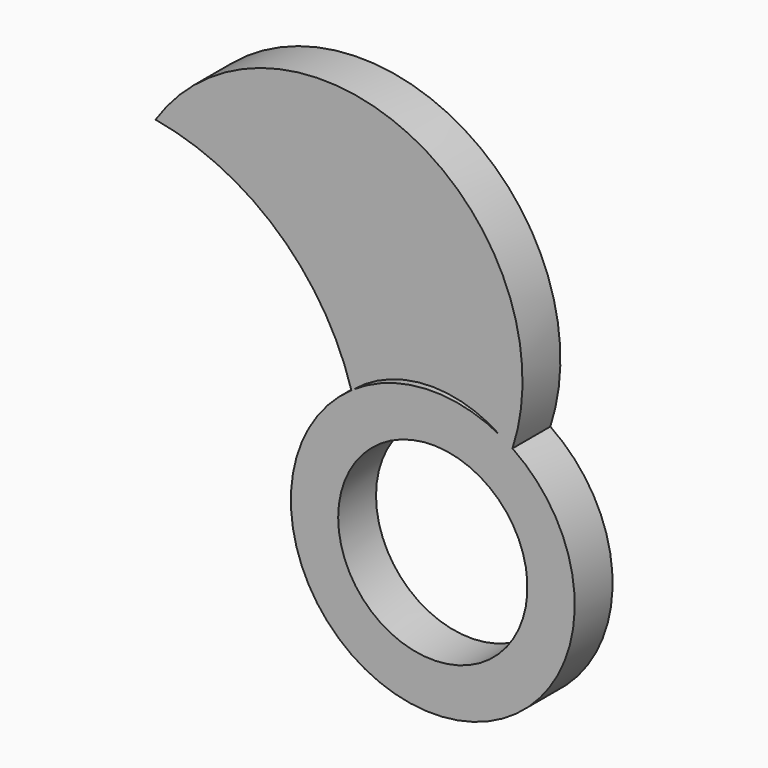
from build123d import *

# Parameters (mm, degrees)
F0_R     = 7.62
F1_DEPTH = 1.27
F3_D     = 10.16
F5_DEPTH = 1.27


# Not quite as in the source:
# - a feature names something its author has since deleted; it is built from what else it names


with BuildPart() as f1:
    # F0 (on Front) → F1 (new body, symmetric)
    with BuildSketch(Plane.XZ):
        Circle(F0_R)
    extrude(amount=F1_DEPTH, both=True)

    # F3 (through all)
    with Locations(Plane.XZ.offset(1.27)):
        with Locations((0, 0)):
            Hole(F3_D / 2)

    # F4 (on Front) → F5 (join, symmetric)
    with BuildSketch(Plane.XZ):
        with BuildLine():
            ThreePointArc((-4.368594382, 6.2292921357), (-0.0581857965, 7.8272864293), (4.2522227889, 6.2292921357))
            ThreePointArc((4.2522227889, 6.2292921357), (-1.1998943931, 19.3169425848), (-14.8855810985, 15.6136797741))
            ThreePointArc((-14.8855810985, 15.6136797741), (-8.2843431722, 12.4262859834), (-4.368594382, 6.2292921357))
        make_face()
    extrude(amount=F5_DEPTH, both=True)


solid = f1.part
